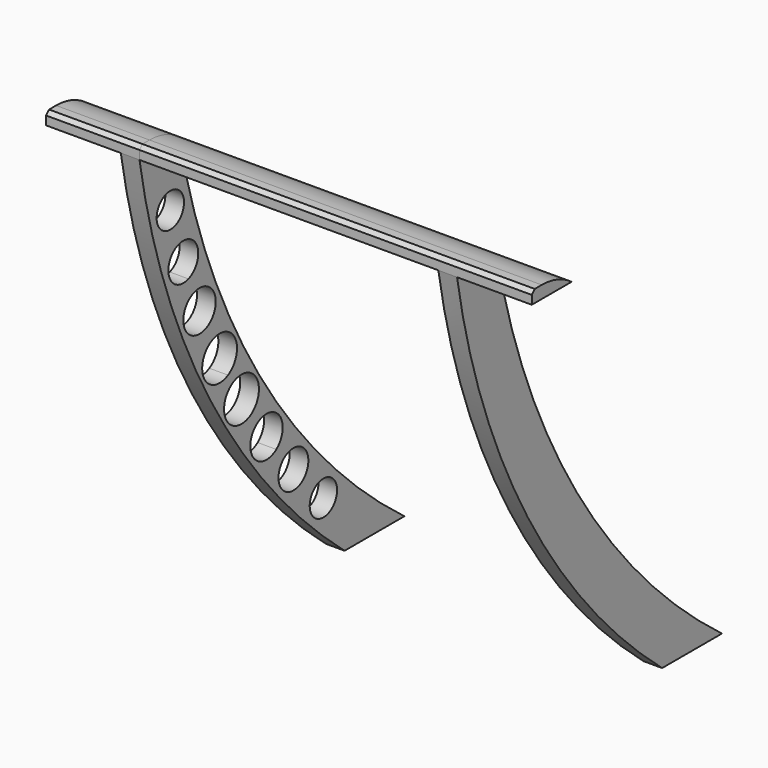
from build123d import *

# Parameters (mm, degrees)
F1_DEPTH      = 38.1
F2_W          = 609.6
F2_H          = 101.6
F2_W_2        = 152.4
F2_W_3        = 38.1
F3_DEPTH      = 25.4
F5_DEPTH      = 38.1
F6_W          = 152.4
F6_H          = 101.6
F6_W_2        = 38.1
F7_DEPTH      = 25.4
F8_T1_DEPTH   = 342.8999998581
F8_T3_DEPTH   = 38.0999997161
F8_T5_DEPTH   = 800.1000004258
F8_2_T1_DEPTH = 571.5
F9_SIZE       = 7.62
F9_2_SIZE     = 7.62
F11_DEPTH     = 762


# Not quite as in the source:
# - a fillet or chamfer that OpenCascade refuses, or shapes differently, is made with other operations: its cross-section is extruded or revolved along the edge and cut away or added


with BuildPart() as f1:
    # F0 (on Right) → F1 (new body)
    with BuildSketch(Plane.YZ):
        with BuildLine():
            Line((-152.4, 0), (0, 0))
            ThreePointArc((0, 0), (-370.5404323347, 404.6996785445), (-573.7339955129, 914.4))
            Line((-573.7339955129, 914.4), (-675.3339955129, 914.4))
            ThreePointArc((-675.3339955129, 914.4), (-495.3809833516, 410.5831647228), (-152.4, 0))
        make_face()
    extrude(amount=F1_DEPTH)

    # F2 (on face) → F3 (join)
    with BuildSketch(Plane.XY.offset(914.4)):
        with Locations((-304.8, -624.5339955129)):
            Rectangle(F2_W, F2_H)
        with Locations((114.3, -624.5339955129)):
            Rectangle(F2_W_2, F2_H)
        with Locations((19.05, -624.5339955129)):
            Rectangle(F2_W_3, F2_H)
    extrude(amount=F3_DEPTH)

    # F8: fillet of radius 127 on 1 edges, made by hand

    # F8_s2 → F8_t1 (cut)
    with BuildSketch(Plane.YZ.offset(38.1000001419)):
        with BuildLine():
            ThreePointArc((-573.7339955129, 914.4), (-609.7730692288, 933.2827788524), (-649.9339955129, 939.8))
            Line((-649.9339955129, 939.8), (-573.7339955129, 939.8))
            Line((-573.7339955129, 939.8), (-573.7339955129, 914.4))
        make_face()
    extrude(amount=F8_T1_DEPTH, mode=Mode.SUBTRACT)

    # F8_s4 → F8_t3 (cut)
    with BuildSketch(Plane.YZ.offset(4.258e-07)):
        with BuildLine():
            ThreePointArc((-573.7339955129, 914.4), (-609.7730692288, 933.2827788524), (-649.9339955129, 939.8))
            Line((-649.9339955129, 939.8), (-573.7339955129, 939.8))
            Line((-573.7339955129, 939.8), (-573.7339955129, 914.4))
        make_face()
    extrude(amount=F8_T3_DEPTH, mode=Mode.SUBTRACT)

    # F8_s6 → F8_t5 (cut)
    with BuildSketch(Plane.YZ.offset(-800.1)):
        with BuildLine():
            ThreePointArc((-573.7339955129, 914.4), (-609.7730692288, 933.2827788524), (-649.9339955129, 939.8))
            Line((-649.9339955129, 939.8), (-573.7339955129, 939.8))
            Line((-573.7339955129, 939.8), (-573.7339955129, 914.4))
        make_face()
    extrude(amount=F8_T5_DEPTH, mode=Mode.SUBTRACT)

    # F9
    f9_edges = [f1.edges().sort_by_distance(p)[0] for p in [
        (-209.55, -675.333996, 939.8),
    ]]
    chamfer(f9_edges, length=F9_SIZE)


with BuildPart() as f5:
    # F4 (on face) → F5 (new body)
    with BuildSketch(Plane(origin=(-609.6, 0, 0), x_dir=(0, -1, 0), z_dir=(-1, 0, 0))):
        with BuildLine():
            Line((675.3339955129, 914.4), (573.7339955129, 914.4))
            ThreePointArc((573.7339955129, 914.4), (370.5404323347, 404.6996785445), (0, 0))
            Line((0, 0), (152.4, 0))
            ThreePointArc((152.4, 0), (495.3809833516, 410.5831647228), (675.3339955129, 914.4))
        make_face()
    extrude(amount=F5_DEPTH)

    # F10 (on face) → F11 (cut)
    with BuildSketch(Plane(origin=(-647.7, 0, 0), x_dir=(0, -1, 0), z_dir=(-1, 0, 0))):
        with BuildLine():
            ThreePointArc((631.5913753294, 792.0699234096), (624.2879152452, 813.4429474745), (605.4321107523, 825.876986392))
            ThreePointArc((605.4321107523, 825.876986392), (596.6663753294, 792.0699234096), (587.1282473408, 758.472605965))
            ThreePointArc((587.1282473408, 758.472605965), (617.7214994682, 764.2052975822), (631.5913753294, 792.0699234096))
        make_face()
        with BuildLine():
            ThreePointArc((587.1282473408, 758.472605965), (596.6663753294, 792.0699234096), (605.4321107523, 825.876986392))
            ThreePointArc((605.4321107523, 825.876986392), (562.9619724604, 801.2224559686), (587.1282473408, 758.472605965))
        make_face()
        with BuildLine():
            ThreePointArc((550.4966543465, 649.9899449451), (563.5869997391, 685.7705662017), (575.778808754, 721.8672390808))
            ThreePointArc((575.778808754, 721.8672390808), (527.6455446354, 698.4126311054), (550.4966543465, 649.9899449451))
        make_face()
        with BuildLine():
            ThreePointArc((601.6869997391, 685.7705662017), (594.5395272891, 707.986574805), (575.778808754, 721.8672390808))
            ThreePointArc((575.778808754, 721.8672390808), (563.5869997391, 685.7705662017), (550.4966543465, 649.9899449451))
            ThreePointArc((550.4966543465, 649.9899449451), (585.4143660546, 654.5427568048), (601.6869997391, 685.7705662017))
        make_face()
        with BuildLine():
            ThreePointArc((563.5267279961, 580.8319471591), (556.6393542578, 603.6599296605), (538.2757632433, 618.869506484))
            ThreePointArc((538.2757632433, 618.869506484), (522.2517279961, 580.8319471591), (505.2034801813, 543.2422827359))
            ThreePointArc((505.2034801813, 543.2422827359), (544.6119515689, 546.1383450576), (563.5267279961, 580.8319471591))
        make_face()
        with BuildLine():
            ThreePointArc((505.2034801813, 543.2422827359), (522.2517279961, 580.8319471591), (538.2757632433, 618.869506484))
            ThreePointArc((538.2757632433, 618.869506484), (484.4346485768, 597.3696050705), (505.2034801813, 543.2422827359))
        make_face()
        with BuildLine():
            ThreePointArc((491.3765799038, 514.6013703621), (471.0563792428, 475.0679421639), (449.5918860193, 436.1439388927))
            ThreePointArc((449.5918860193, 436.1439388927), (493.658434196, 436.793281984), (515.5063792428, 475.0679421639))
            ThreePointArc((515.5063792428, 475.0679421639), (508.9973558998, 498.2257656867), (491.3765799038, 514.6013703621))
        make_face()
        with BuildLine():
            ThreePointArc((491.3765799038, 514.6013703621), (431.8234913863, 495.962511086), (449.5918860193, 436.1439388927))
            ThreePointArc((449.5918860193, 436.1439388927), (471.0563792428, 475.0679421639), (491.3765799038, 514.6013703621))
        make_face()
        with BuildLine():
            ThreePointArc((438.3828882756, 416.8305093134), (377.6291498002, 402.5840820999), (390.9880699941, 341.6290439297))
            ThreePointArc((390.9880699941, 341.6290439297), (415.2338814717, 378.8841526504), (438.3828882756, 416.8305093134))
        make_face()
        with BuildLine():
            ThreePointArc((438.3828882756, 416.8305093134), (415.2338814717, 378.8841526504), (390.9880699941, 341.6290439297))
            ThreePointArc((390.9880699941, 341.6290439297), (436.4244003401, 339.8103198452), (459.6838814717, 378.8841526504))
            ThreePointArc((459.6838814717, 378.8841526504), (453.9945306693, 400.6422447953), (438.3828882756, 416.8305093134))
        make_face()
        with BuildLine():
            ThreePointArc((375.559494086, 319.1005287315), (351.4771368764, 285.5794055964), (326.4958314478, 252.7227471528))
            ThreePointArc((326.4958314478, 252.7227471528), (369.8145609517, 248.6015135083), (392.7521368764, 285.5794055964))
            ThreePointArc((392.7521368764, 285.5794055964), (388.2033190822, 304.4158905549), (375.559494086, 319.1005287315))
        make_face()
        with BuildLine():
            ThreePointArc((307.2689413413, 228.6388188544), (253.9087320552, 224.2096185946), (257.6705836541, 170.7982132344))
            ThreePointArc((257.6705836541, 170.7982132344), (282.8312945287, 199.4085020881), (307.2689413413, 228.6388188544))
        make_face()
        with BuildLine():
            ThreePointArc((307.2689413413, 228.6388188544), (282.8312945287, 199.4085020881), (257.6705836541, 170.7982132344))
            ThreePointArc((257.6705836541, 170.7982132344), (298.5314046506, 164.6937135656), (320.9312945287, 199.4085020881))
            ThreePointArc((320.9312945287, 199.4085020881), (317.3471194758, 215.5413204475), (307.2689413413, 228.6388188544))
        make_face()
        with BuildLine():
            ThreePointArc((375.559494086, 319.1005287315), (318.2852026333, 310.1134865085), (326.4958314478, 252.7227471528))
            ThreePointArc((326.4958314478, 252.7227471528), (351.4771368764, 285.5794055964), (375.559494086, 319.1005287315))
        make_face()
        with BuildLine():
            ThreePointArc((230.7606464602, 141.7281596434), (181.6547503588, 141.316474077), (181.5037371724, 92.2090844911))
            ThreePointArc((181.5037371724, 92.2090844911), (206.4159134771, 116.686402497), (230.7606464602, 141.7281596434))
        make_face()
        with BuildLine():
            ThreePointArc((230.7606464602, 141.7281596434), (206.4159134771, 116.686402497), (181.5037371724, 92.2090844911))
            ThreePointArc((181.5037371724, 92.2090844911), (219.6389590332, 84.3613860049), (241.3409134771, 116.686402497))
            ThreePointArc((241.3409134771, 116.686402497), (238.5872938052, 130.2789707894), (230.7606464602, 141.7281596434))
        make_face()
    extrude(amount=-F11_DEPTH, mode=Mode.SUBTRACT)


with BuildPart() as f7:
    # F6 (on face) → F7 (new body)
    with BuildSketch(Plane.XY.offset(914.4)):
        with Locations((-723.9, -624.5339955129)):
            Rectangle(F6_W, F6_H)
        with Locations((-628.65, -624.5339955129)):
            Rectangle(F6_W_2, F6_H)
    extrude(amount=F7_DEPTH)

    # F8#2: fillet of radius 127 on 1 edges, made by hand

    # F8_2_s2 → F8_2_t1 (cut)
    with BuildSketch(Plane.YZ.offset(-990.6)):
        with BuildLine():
            ThreePointArc((-573.7339955129, 914.4), (-609.7730692288, 933.2827788524), (-649.9339955129, 939.8))
            Line((-649.9339955129, 939.8), (-573.7339955129, 939.8))
            Line((-573.7339955129, 939.8), (-573.7339955129, 914.4))
        make_face()
    extrude(amount=F8_2_T1_DEPTH, mode=Mode.SUBTRACT)

    # F9#2
    f9_2_edges = [f7.edges().sort_by_distance(p)[0] for p in [
        (-704.85, -675.333996, 939.8),
    ]]
    chamfer(f9_2_edges, length=F9_2_SIZE)


solid = Compound([f1.part, f5.part, f7.part])
